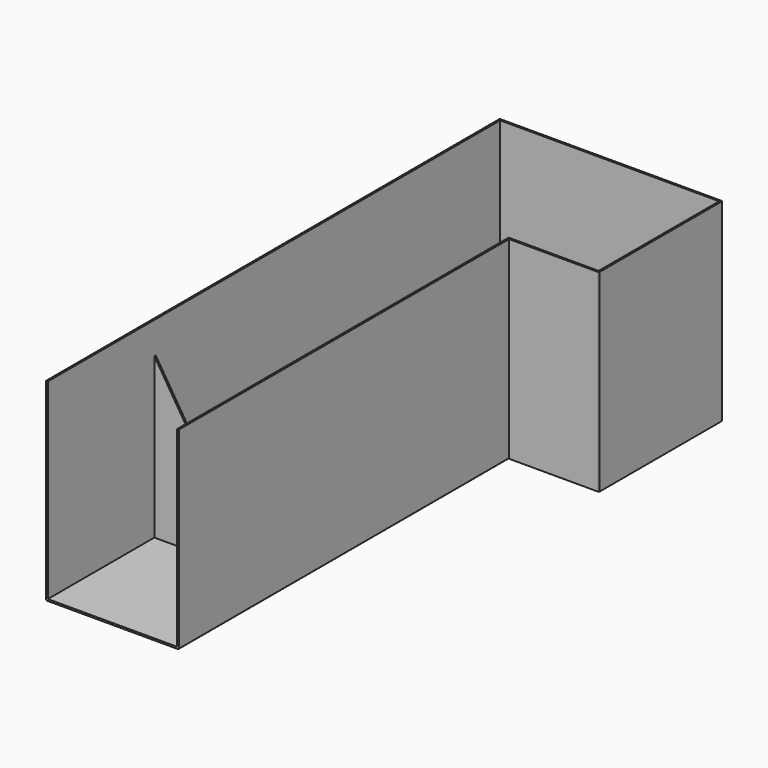
from build123d import *

# Parameters (mm, degrees)
F1_DEPTH  = 426
F3_DEPTH  = 4
F4_R      = 2
F7_DEPTH  = 4
F10_DEPTH = 4


# Not quite as in the source:
# - a feature names something its author has since deleted; it is built from what else it names


with BuildPart() as f1:
    # F0 (on Top) → F1 (new body)
    with BuildSketch(Plane.XY):
        Polygon((-200, -343), (0, -343), (0, 0), (-495, 0), (-495, -1261), (-491, -1261), (-491, -4), (-4, -4), (-4, -339), (-204, -339), (-204, -1261), (-200, -1261), align=None)
    extrude(amount=F1_DEPTH)

    # F2 (on Top) → F3 (join)
    with BuildSketch(Plane.XY):
        Polygon((0, 0), (-495, 0), (-495, -1261), (-200, -1261), (-200, -343), (0, -343), align=None)
    extrude(amount=-F3_DEPTH)

    # F4
    f4_edges = [f1.edges().sort_by_distance(p)[0] for p in [
        (-200, -802, -4),
        (-495, -630.5, -4),
        (-247.5, 0, -4),
        (0, -343, 211),
        (0, 0, 211),
    ]]
    fillet(f4_edges, radius=F4_R)

    # F6 (on offset) → F7 (join)
    with BuildSketch(Plane.XZ.offset(961)):
        Polygon((-491, 355), (-491, 0), (-269, 0), align=None)
    extrude(amount=F7_DEPTH)

    # F9 (on offset) → F10 (join)
    with BuildSketch(Plane.XZ.offset(361)):
        Polygon((-426, 0), (-204, 0), (-204, 355), align=None)
    extrude(amount=F10_DEPTH)


solid = f1.part
